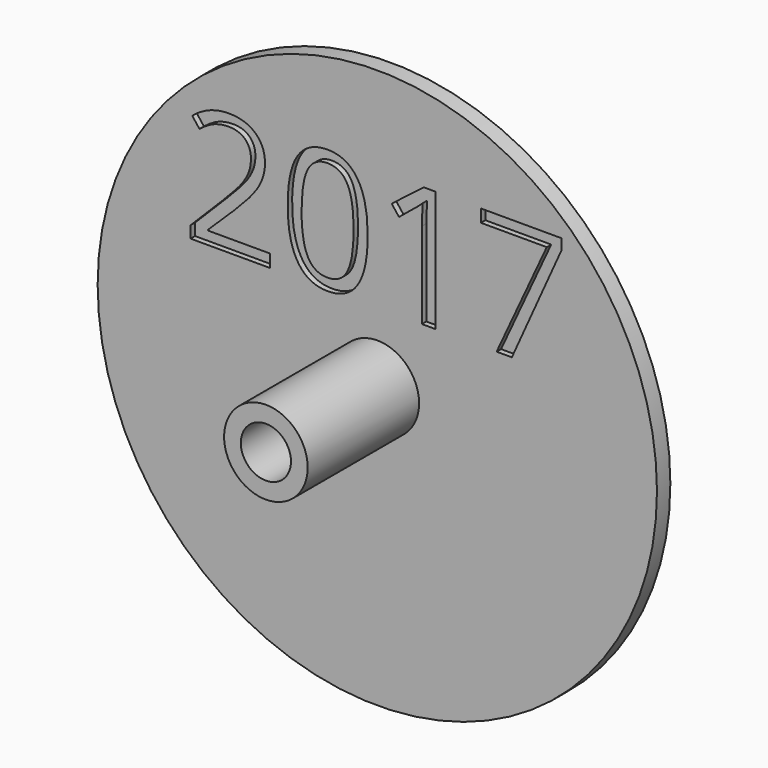
from build123d import *

# Parameters (mm, degrees)
F0_R         = 50.2
F0_R_2       = 4.5
F1_DEPTH     = 3
F2_R         = 7.5
F2_R_2       = 4.5
F3_DEPTH     = 25
F4_TEXT_SIZE = 30.4223821812
F5_DEPTH     = 1


# Not quite as in the source:
# - Text() gives the source's letters only with a copy of the font that has no kerning and outlines rounded to 1/6400 em; it was checked with that copy


with BuildPart() as f1:
    # F0 (on Front) → F1 (new body)
    with BuildSketch(Plane.XZ):
        Circle(F0_R)
        Circle(F0_R_2, mode=Mode.SUBTRACT)
    extrude(amount=F1_DEPTH)

    # F2 (on face) → F3 (join)
    with BuildSketch(Plane.XZ.offset(3)):
        Circle(F2_R)
        Circle(F2_R_2, mode=Mode.SUBTRACT)
    extrude(amount=F3_DEPTH)

    # F4 (on face) → F5 (cut)
    with BuildSketch(Plane.XZ.offset(3)):
        with Locations((-35, 12.6814708964)):
            Text('2017', F4_TEXT_SIZE, font='Open Sans', text_align=(TextAlign.LEFT, TextAlign.BOTTOM))
    extrude(amount=-F5_DEPTH, mode=Mode.SUBTRACT)


solid = f1.part
